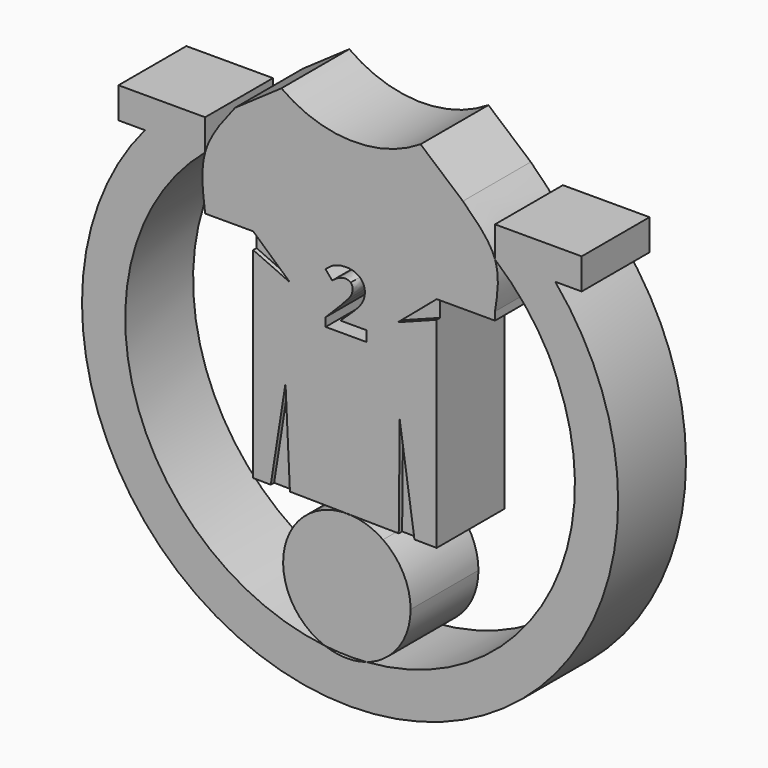
from build123d import *

# Parameters (mm, degrees)
F1_DEPTH = 7.62
F2_DEPTH = 7.239


# Not quite as in the source:
# - the program builds the solid bodies; features that only make, move or delete a surface that nothing else refers to are left out


with BuildPart() as f1:
    # F0 (on Front) → F1 (new body)
    with BuildSketch(Plane.XZ):
        with BuildLine():
            Line((-59.5584991262, 48.2375602462), (-64.9708399911, 48.2375602462))
            ThreePointArc((-64.9708399911, 48.2375602462), (-46.5380060703, 8.6596191309), (-28.1051721496, 48.2375602462))
            Line((-28.1051721496, 48.2375602462), (-33.5175130144, 48.2375602462))
            ThreePointArc((-33.5175130144, 48.2375602462), (-27.3247565054, 26.5574116364), (-45.0697709813, 12.6472161608))
            ThreePointArc((-45.0697709813, 12.6472161608), (-46.9391212719, 12.3720803787), (-48.7962257348, 12.7204095643))
            ThreePointArc((-48.7962257348, 12.7204095643), (-65.87002003, 26.9359197848), (-59.5584991262, 48.2375602462))
        make_face()
        Polygon((-67.3419212263, 48.2375602462), (-64.9708399911, 48.2375602462), (-59.5584991262, 48.2375602462), (-59.5584991262, 51.0173538534), (-67.3419212263, 51.0173538534), align=None)
        Polygon((-33.5175130144, 48.2375602462), (-28.1051721496, 48.2375602462), (-25.7340909143, 48.2375602462), (-25.7340909143, 51.0173538534), (-33.5175130144, 51.0173538534), align=None)
    extrude(amount=F1_DEPTH)


with BuildPart() as f1b:
    # F0 (on Front) → F1, piece 2 (new body)
    with BuildSketch(Plane.XZ):
        with BuildLine():
            add(Edge.make_bspline(
                [(-56.8707543748, 52.6390547806), (-57.9942418052, 51.2220877516), (-59.1177292355, 49.8051207226), (-59.5584991262, 48.2375602462)],
                knots=[0, 0, 0, 0, 0.5080226009, 0.5080226009, 0.5080226009, 0.5080226009], degree=3))
            add(Edge.make_bspline(
                [(-59.5584991262, 48.2375602462), (-59.9853479003, 46.7195090321), (-59.7719235132, 45.0602267275), (-59.5584991262, 43.4009444229)],
                knots=[0.5080226009, 0.5080226009, 0.5080226009, 0.5080226009, 1, 1, 1, 1], degree=3))
            Line((-59.5584991262, 43.4009444229), (-55.2404991262, 43.4009444229))
            Line((-55.2404991262, 43.4009444229), (-51.9395383562, 40.4397919774))
            Line((-51.9395383562, 40.4397919774), (-55.2404991262, 41.9203682002))
            Line((-55.2404991262, 41.9203682002), (-55.2404991262, 23.888412863))
            Line((-55.2404991262, 23.888412863), (-53.664046478, 23.8725836956))
            Line((-53.664046478, 23.8725836956), (-52.338115871, 32.3296152055))
            Line((-52.338115871, 32.3296152055), (-51.9395383562, 23.888412863))
            Line((-51.9395383562, 23.888412863), (-46.7522454605, 23.8209567953))
            Line((-46.7522454605, 23.8209567953), (-42.1669552674, 23.7613292301))
            Line((-42.1669552674, 23.7613292301), (-42.0762598515, 32.7938339318))
            Line((-42.0762598515, 32.7938339318), (-40.753610712, 23.7429499583))
            Line((-40.753610712, 23.7429499583), (-38.7568103386, 23.7229000777))
            Line((-38.7568103386, 23.7229000777), (-38.7568103386, 41.7639017105))
            Line((-38.7568103386, 41.7639017105), (-42.2417744994, 40.4397919774))
            Line((-42.2417744994, 40.4397919774), (-38.7568103386, 43.4009444229))
            Line((-38.7568103386, 43.4009444229), (-33.5175130144, 43.4009444229))
            Line((-33.5175130144, 43.4009444229), (-33.5175130144, 44.1255018582))
            add(Edge.make_bspline(
                [(-33.5175130144, 48.2375602462), (-33.0809784188, 46.9738387084), (-33.2992457166, 45.5496702833), (-33.5175130144, 44.1255018582)],
                knots=[0.5159883661, 0.5159883661, 0.5159883661, 0.5159883661, 1, 1, 1, 1], degree=3))
            add(Edge.make_bspline(
                [(-36.4019976546, 51.9144973453), (-35.1924426885, 50.7496341038), (-33.9828877223, 49.5847708622), (-33.5175130144, 48.2375602462)],
                knots=[0, 0, 0, 0, 0.5159883661, 0.5159883661, 0.5159883661, 0.5159883661], degree=3))
            Line((-36.4019976546, 51.9144973453), (-40.2059252092, 55.1750078426))
            ThreePointArc((-40.2059252092, 55.1750078426), (-46.5111214901, 53.4280963412), (-52.7045460642, 55.5372885988))
            Line((-52.7045460642, 55.5372885988), (-56.8707543748, 52.6390547806))
        make_face()
        with BuildLine():
            Line((-45.0624059546, 38.8915469496), (-45.0624059546, 37.9570834339))
            Line((-45.0624059546, 37.9570834339), (-48.7335947239, 37.9570834339))
            Line((-48.7335947239, 37.9570834339), (-48.7335947239, 38.7294813214))
            Line((-48.7335947239, 38.7294813214), (-47.4152310675, 40.0616377972))
            add(Edge.make_bspline(
                [(-47.4152310675, 40.0616377972), (-46.8290362421, 40.661625442), (-46.6497295897, 40.8932298681)],
                knots=[0, 0, 0, 1, 1, 1], degree=2))
            add(Edge.make_bspline(
                [(-46.6497295897, 40.8932298681), (-46.4704229372, 41.1248342942), (-46.3911142255, 41.3225313726)],
                knots=[0, 0, 0, 1, 1, 1], degree=2))
            add(Edge.make_bspline(
                [(-46.3911142255, 41.3225313726), (-46.3118055138, 41.520228451), (-46.3118055138, 41.7317183488)],
                knots=[0, 0, 0, 1, 1, 1], degree=2))
            add(Edge.make_bspline(
                [(-46.3118055138, 41.7317183488), (-46.3118055138, 42.0478037938), (-46.4865145598, 42.2023983115)],
                knots=[0, 0, 0, 1, 1, 1], degree=2))
            add(Edge.make_bspline(
                [(-46.4865145598, 42.2023983115), (-46.6612236059, 42.3569928292), (-46.9520222153, 42.3569928292)],
                knots=[0, 0, 0, 1, 1, 1], degree=2))
            add(Edge.make_bspline(
                [(-46.9520222153, 42.3569928292), (-47.2566136442, 42.3569928292), (-47.5439640488, 42.2167658318)],
                knots=[0, 0, 0, 1, 1, 1], degree=2))
            add(Edge.make_bspline(
                [(-47.5439640488, 42.2167658318), (-47.8313144534, 42.0765388343), (-48.1439516936, 41.8179234702)],
                knots=[0, 0, 0, 1, 1, 1], degree=2))
            Line((-48.1439516936, 41.8179234702), (-48.7473875433, 42.5328512768))
            add(Edge.make_bspline(
                [(-48.7473875433, 42.5328512768), (-48.3600391979, 42.8638789429), (-48.1048720386, 43.0000830347)],
                knots=[0, 0, 0, 1, 1, 1], degree=2))
            add(Edge.make_bspline(
                [(-48.1048720386, 43.0000830347), (-47.8497048793, 43.1362871265), (-47.5479869545, 43.2098488301)],
                knots=[0, 0, 0, 1, 1, 1], degree=2))
            add(Edge.make_bspline(
                [(-47.5479869545, 43.2098488301), (-47.2462690296, 43.2834105337), (-46.8727135036, 43.2834105337)],
                knots=[0, 0, 0, 1, 1, 1], degree=2))
            add(Edge.make_bspline(
                [(-46.8727135036, 43.2834105337), (-46.380769611, 43.2834105337), (-46.0037658801, 43.1041038812)],
                knots=[0, 0, 0, 1, 1, 1], degree=2))
            add(Edge.make_bspline(
                [(-46.0037658801, 43.1041038812), (-45.6267621493, 42.9247972287), (-45.4181457555, 42.6012406731)],
                knots=[0, 0, 0, 1, 1, 1], degree=2))
            add(Edge.make_bspline(
                [(-45.4181457555, 42.6012406731), (-45.2095293618, 42.2776841175), (-45.2095293618, 41.8616007317)],
                knots=[0, 0, 0, 1, 1, 1], degree=2))
            add(Edge.make_bspline(
                [(-45.2095293618, 41.8616007317), (-45.2095293618, 41.4983898202), (-45.3371129414, 41.1805802727)],
                knots=[0, 0, 0, 1, 1, 1], degree=2))
            add(Edge.make_bspline(
                [(-45.3371129414, 41.1805802727), (-45.4646965211, 40.8627707252), (-45.7325070982, 40.5288695551)],
                knots=[0, 0, 0, 1, 1, 1], degree=2))
            add(Edge.make_bspline(
                [(-45.7325070982, 40.5288695551), (-46.0003176753, 40.1949683849), (-46.6750164253, 39.5765903142)],
                knots=[0, 0, 0, 1, 1, 1], degree=2))
            Line((-46.6750164253, 39.5765903142), (-47.3508645769, 38.9409712192))
            Line((-47.3508645769, 38.9409712192), (-47.3508645769, 38.8915469496))
            Line((-47.3508645769, 38.8915469496), (-45.0624059546, 38.8915469496))
        make_face(mode=Mode.SUBTRACT)
    extrude(amount=F1_DEPTH)

    # F0 (on Front) → F2 (join)
    with BuildSketch(Plane.XZ):
        with BuildLine():
            Line((-53.664046478, 23.8725836956), (-47.2204577548, 23.8078835954))
            ThreePointArc((-47.2204577548, 23.8078835954), (-46.9864853573, 23.8192103943), (-46.7522454605, 23.8209567953))
            Line((-46.7522454605, 23.8209567953), (-51.9395383562, 23.888412863))
            Line((-51.9395383562, 23.888412863), (-52.338115871, 32.3296152055))
            Line((-52.338115871, 32.3296152055), (-53.664046478, 23.8725836956))
        make_face()
        Polygon((-42.1669552674, 23.7613292301), (-40.753610712, 23.7429499583), (-42.0762598515, 32.7938339318), align=None)
        Polygon((-51.9395383562, 40.4397919774), (-55.2404991262, 43.4009444229), (-55.2404991262, 41.9203682002), align=None)
        Polygon((-38.7568103386, 41.7639017105), (-38.7568103386, 43.4009444229), (-42.2417744994, 40.4397919774), align=None)
    extrude(amount=F2_DEPTH)


with BuildPart() as f1c:
    # F0 (on Front) → F1, piece 3 (new body)
    with BuildSketch(Plane.XZ):
        with BuildLine():
            ThreePointArc((-49.9709981221, 13.3116904732), (-49.4006466899, 12.9822049089), (-48.7962257348, 12.7204095643))
            ThreePointArc((-48.7962257348, 12.7204095643), (-46.9346901082, 12.5976817324), (-45.0697709813, 12.6472161608))
            ThreePointArc((-45.0697709813, 12.6472161608), (-44.3242339331, 12.9468400942), (-43.6279851846, 13.3478858171))
            ThreePointArc((-43.6279851846, 13.3478858171), (-43.7477560192, 13.547239909), (-43.8622818599, 13.7496527016))
            ThreePointArc((-43.8622818599, 13.7496527016), (-44.0069124158, 14.0244973728), (-44.141874165, 14.3042167273))
            ThreePointArc((-44.141874165, 14.3042167273), (-44.2788871247, 14.6169348112), (-44.4038162039, 14.9346735031))
            ThreePointArc((-44.4038162039, 14.9346735031), (-44.524631527, 15.2819339234), (-44.6310139513, 15.6338840926))
            ThreePointArc((-44.6310139513, 15.6338840926), (-44.7241488842, 15.9957276415), (-44.8020281543, 16.3611584679))
            ThreePointArc((-44.8020281543, 16.3611584679), (-44.8689286768, 16.7596883146), (-44.917686063, 17.1608421952))
            ThreePointArc((-44.917686063, 17.1608421952), (-44.9461032037, 17.5257356006), (-44.9595074387, 17.8914883281))
            ThreePointArc((-44.9595074387, 17.8914883281), (-44.9587241846, 18.2204976343), (-44.945791906, 18.5492536124))
            ThreePointArc((-44.945791906, 18.5492536124), (-44.9154647205, 18.9309840033), (-44.8687597947, 19.311058311))
            ThreePointArc((-44.8687597947, 19.311058311), (-44.7993413756, 19.7224063942), (-44.7107409222, 20.13005345))
            ThreePointArc((-44.7107409222, 20.13005345), (-44.6269832671, 20.4500506858), (-44.5314031498, 20.7667177299))
            ThreePointArc((-44.5314031498, 20.7667177299), (-44.4182724978, 21.0956811982), (-44.292384048, 21.4199767518))
            ThreePointArc((-44.292384048, 21.4199767518), (-44.1668612228, 21.7106973118), (-44.0310848775, 21.9967728398))
            ThreePointArc((-44.0310848775, 21.9967728398), (-43.9091335777, 22.2334098214), (-43.7801657509, 22.4662970908))
            ThreePointArc((-43.7801657509, 22.4662970908), (-43.6790232251, 22.6381795939), (-43.5740581992, 22.8077547948))
            ThreePointArc((-43.5740581992, 22.8077547948), (-44.8819912009, 23.4810418249), (-46.3183121682, 23.7988251479))
            Line((-46.3183121682, 23.7988251479), (-47.2204577548, 23.8078835954))
            ThreePointArc((-47.2204577548, 23.8078835954), (-48.4659781229, 23.5817368193), (-49.631357065, 23.0874137743))
            ThreePointArc((-49.631357065, 23.0874137743), (-49.4399703042, 22.8012645954), (-49.2608678419, 22.507270458))
            ThreePointArc((-49.2608678419, 22.507270458), (-49.0909371231, 22.1994140873), (-48.934476517, 21.8844981097))
            ThreePointArc((-48.934476517, 21.8844981097), (-48.7796011354, 21.533843634), (-48.6414253274, 21.1762791067))
            ThreePointArc((-48.6414253274, 21.1762791067), (-48.5264267045, 20.8325949559), (-48.4268576249, 20.4841276301))
            ThreePointArc((-48.4268576249, 20.4841276301), (-48.3512675692, 20.1700219292), (-48.2882156381, 19.8531612313))
            ThreePointArc((-48.2882156381, 19.8531612313), (-48.2364890834, 19.5244720475), (-48.1982539758, 19.1939417273))
            ThreePointArc((-48.1982539758, 19.1939417273), (-48.1743949079, 18.8771098565), (-48.1629326852, 18.5595877205))
            ThreePointArc((-48.1629326852, 18.5595877205), (-48.1640132648, 18.2362473997), (-48.1779489959, 17.9132057212))
            ThreePointArc((-48.1779489959, 17.9132057212), (-48.200015614, 17.6379014311), (-48.2314197618, 17.3635054266))
            ThreePointArc((-48.2314197618, 17.3635054266), (-48.2744314156, 17.0765495957), (-48.3276546289, 16.7913112028))
            ThreePointArc((-48.3276546289, 16.7913112028), (-48.4096419855, 16.4329658061), (-48.5077428192, 16.0786924987))
            ThreePointArc((-48.5077428192, 16.0786924987), (-48.5962780883, 15.8028375106), (-48.6945848527, 15.5303118267))
            ThreePointArc((-48.6945848527, 15.5303118267), (-48.807250429, 15.2503283661), (-48.9302291917, 14.9747190516))
            ThreePointArc((-48.9302291917, 14.9747190516), (-49.0672773505, 14.6962471277), (-49.2148536279, 14.4232085726))
            ThreePointArc((-49.2148536279, 14.4232085726), (-49.341263487, 14.2074529376), (-49.4742483135, 13.9956865985))
            ThreePointArc((-49.4742483135, 13.9956865985), (-49.6022091028, 13.8046791412), (-49.7355192028, 13.6173659555))
            ThreePointArc((-49.7355192028, 13.6173659555), (-49.8514451058, 13.4631311302), (-49.9709981221, 13.3116904732))
        make_face()
        with BuildLine():
            ThreePointArc((-49.631357065, 23.0874137743), (-52.5484703481, 18.2950021878), (-49.9709981221, 13.3116904732))
            ThreePointArc((-49.9709981221, 13.3116904732), (-49.8514451058, 13.4631311302), (-49.7355192028, 13.6173659555))
            ThreePointArc((-49.7355192028, 13.6173659555), (-49.6022091028, 13.8046791412), (-49.4742483135, 13.9956865985))
            ThreePointArc((-49.4742483135, 13.9956865985), (-49.341263487, 14.2074529376), (-49.2148536279, 14.4232085726))
            ThreePointArc((-49.2148536279, 14.4232085726), (-49.0672773505, 14.6962471277), (-48.9302291917, 14.9747190516))
            ThreePointArc((-48.9302291917, 14.9747190516), (-48.807250429, 15.2503283661), (-48.6945848527, 15.5303118267))
            ThreePointArc((-48.6945848527, 15.5303118267), (-48.5962780883, 15.8028375106), (-48.5077428192, 16.0786924987))
            ThreePointArc((-48.5077428192, 16.0786924987), (-48.4096419855, 16.4329658061), (-48.3276546289, 16.7913112028))
            ThreePointArc((-48.3276546289, 16.7913112028), (-48.2744314156, 17.0765495957), (-48.2314197618, 17.3635054266))
            ThreePointArc((-48.2314197618, 17.3635054266), (-48.200015614, 17.6379014311), (-48.1779489959, 17.9132057212))
            ThreePointArc((-48.1779489959, 17.9132057212), (-48.1640132648, 18.2362473997), (-48.1629326852, 18.5595877205))
            ThreePointArc((-48.1629326852, 18.5595877205), (-48.1743949079, 18.8771098565), (-48.1982539758, 19.1939417273))
            ThreePointArc((-48.1982539758, 19.1939417273), (-48.2364890834, 19.5244720475), (-48.2882156381, 19.8531612313))
            ThreePointArc((-48.2882156381, 19.8531612313), (-48.3512675692, 20.1700219292), (-48.4268576249, 20.4841276301))
            ThreePointArc((-48.4268576249, 20.4841276301), (-48.5264267045, 20.8325949559), (-48.6414253274, 21.1762791067))
            ThreePointArc((-48.6414253274, 21.1762791067), (-48.7796011354, 21.533843634), (-48.934476517, 21.8844981097))
            ThreePointArc((-48.934476517, 21.8844981097), (-49.0909371231, 22.1994140873), (-49.2608678419, 22.507270458))
            ThreePointArc((-49.2608678419, 22.507270458), (-49.4399703042, 22.8012645954), (-49.631357065, 23.0874137743))
        make_face()
        with BuildLine():
            ThreePointArc((-43.8622818599, 13.7496527016), (-43.7477560192, 13.547239909), (-43.6279851846, 13.3478858171))
            ThreePointArc((-43.6279851846, 13.3478858171), (-41.7724043969, 15.4068820932), (-41.1014581894, 18.0962085724))
            ThreePointArc((-41.1014581894, 18.0962085724), (-41.7571559778, 20.7566793303), (-43.5740581992, 22.8077547948))
            ThreePointArc((-43.5740581992, 22.8077547948), (-43.6790232251, 22.6381795939), (-43.7801657509, 22.4662970908))
            ThreePointArc((-43.7801657509, 22.4662970908), (-43.9091335777, 22.2334098214), (-44.0310848775, 21.9967728398))
            ThreePointArc((-44.0310848775, 21.9967728398), (-44.1668612228, 21.7106973118), (-44.292384048, 21.4199767518))
            ThreePointArc((-44.292384048, 21.4199767518), (-44.4182724978, 21.0956811982), (-44.5314031498, 20.7667177299))
            ThreePointArc((-44.5314031498, 20.7667177299), (-44.6269832671, 20.4500506858), (-44.7107409222, 20.13005345))
            ThreePointArc((-44.7107409222, 20.13005345), (-44.7993413756, 19.7224063942), (-44.8687597947, 19.311058311))
            ThreePointArc((-44.8687597947, 19.311058311), (-44.9154647205, 18.9309840033), (-44.945791906, 18.5492536124))
            ThreePointArc((-44.945791906, 18.5492536124), (-44.9587241846, 18.2204976343), (-44.9595074387, 17.8914883281))
            ThreePointArc((-44.9595074387, 17.8914883281), (-44.9461032037, 17.5257356006), (-44.917686063, 17.1608421952))
            ThreePointArc((-44.917686063, 17.1608421952), (-44.8689286768, 16.7596883146), (-44.8020281543, 16.3611584679))
            ThreePointArc((-44.8020281543, 16.3611584679), (-44.7241488842, 15.9957276415), (-44.6310139513, 15.6338840926))
            ThreePointArc((-44.6310139513, 15.6338840926), (-44.524631527, 15.2819339234), (-44.4038162039, 14.9346735031))
            ThreePointArc((-44.4038162039, 14.9346735031), (-44.2788871247, 14.6169348112), (-44.141874165, 14.3042167273))
            ThreePointArc((-44.141874165, 14.3042167273), (-44.0069124158, 14.0244973728), (-43.8622818599, 13.7496527016))
        make_face()
    extrude(amount=F1_DEPTH)


solid = Compound([f1.part, f1b.part, f1c.part])
